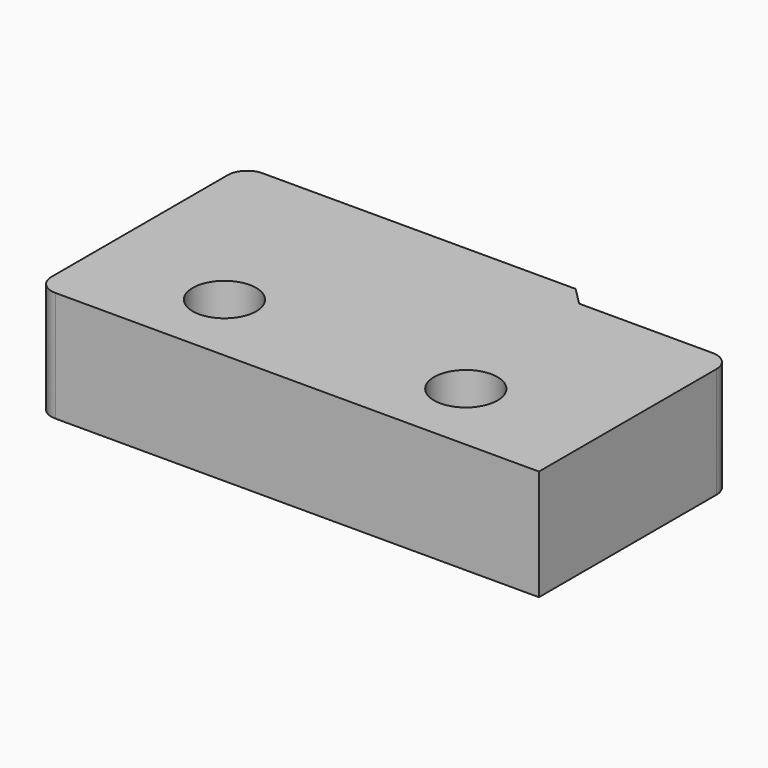
from build123d import *

# Parameters (mm, degrees)
F0_W     = 0.5
F0_H     = 3.5
F0_R     = 1.25
F1_DEPTH = 4.3564048
F2_R     = 0.762
F3_W     = 19.038
F3_H     = 6.3
F3_H_2   = 3.5
F4_DEPTH = 4.3564048


with BuildPart() as f1:
    # F0 (on Top) → F1 (new body)
    with BuildSketch(Plane.XY):
        with Locations((4.1668843009, -11.25)):
            Rectangle(F0_W, F0_H)
        with Locations((-3.3831156991, -11.25)):
            Rectangle(F0_W, F0_H)
        with Locations((-11.9331156991, -11.25)):
            Rectangle(F0_W, F0_H)
        with BuildLine():
            Line((-10.6081156991, 0.7), (-9.8143656991, 0.7))
            Line((-9.8143656991, 0.7), (-9.8143656991, 1.101979753))
            ThreePointArc((-9.8143656991, 1.101979753), (-9.7252470071, 1.317131308), (-9.5100954521, 1.40625))
            Line((-9.5100954521, 1.40625), (6.0168843009, 1.40625))
            Line((6.0168843009, 1.40625), (6.0168843009, 2.2))
            Line((6.0168843009, 2.2), (6.0168843009, 4.6))
            ThreePointArc((6.0168843009, 4.6), (3.6168843009, 7), (1.2168843009, 4.6))
            Line((1.2168843009, 4.6), (1.2168843009, 2.2))
            Line((1.2168843009, 2.2), (-9.5100954521, 2.2))
            ThreePointArc((-9.5100954521, 2.2), (-10.2865130147, 1.8783973155), (-10.6081156991, 1.101979753))
            Line((-10.6081156991, 1.101979753), (-10.6081156991, 0.7))
        make_face()
        with BuildLine():
            Line((6.0168843009, 0), (0, 0))
            Line((0, 0), (-0.7, 0.7))
            Line((-0.7, 0.7), (-5.9126656991, 0.7))
            ThreePointArc((-5.9126656991, 0.7), (-6.5935156991, 1.38085), (-7.2743656991, 0.7))
            Line((-7.2743656991, 0.7), (-9.8143656991, 0.7))
            Line((-9.8143656991, 0.7), (-10.6081156991, 0.7))
            Line((-10.6081156991, 0.7), (-13.7831156991, 0.7))
            Line((-13.7831156991, 0.7), (-13.7831156991, -9.5))
            Line((-13.7831156991, -9.5), (-12.1831156991, -9.5))
            Line((-12.1831156991, -9.5), (-11.6831156991, -9.5))
            Line((-11.6831156991, -9.5), (-3.6331156991, -9.5))
            Line((-3.6331156991, -9.5), (-3.1331156991, -9.5))
            Line((-3.1331156991, -9.5), (3.9168843009, -9.5))
            Line((3.9168843009, -9.5), (4.4168843009, -9.5))
            Line((4.4168843009, -9.5), (6.0168843009, -9.5))
            Line((6.0168843009, -9.5), (6.0168843009, 0))
        make_face()
        with Locations((-8.6831156991, -6.6)):
            Circle(F0_R, mode=Mode.SUBTRACT)
        with Locations((0.8168843009, -6.6)):
            Circle(F0_R, mode=Mode.SUBTRACT)
    extrude(amount=F1_DEPTH)

    # F2
    f2_edges = [f1.edges().sort_by_distance(p)[0] for p in [
        (6.016884, 0, 2.178202),
        (-13.783116, -9.5, 2.178202),
        (-13.783116, 0.7, 2.178202),
    ]]
    fillet(f2_edges, radius=F2_R)

    # F3 (on face) → F4 (cut, through all)
    with BuildSketch(Plane.XY.offset(4.3564048)):
        with Locations((-3.5021156991, 3.85)):
            Rectangle(F3_W, F3_H)
        with Locations((-3.5021156991, -11.25)):
            Rectangle(F3_W, F3_H_2)
    extrude(amount=-F4_DEPTH, mode=Mode.SUBTRACT)


solid = f1.part
